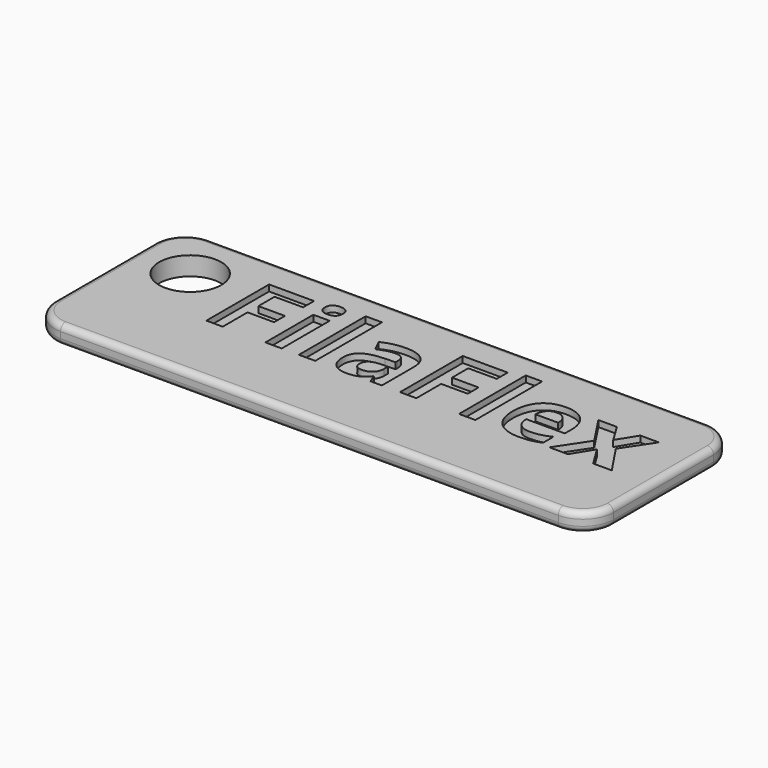
from build123d import *

# Parameters (mm, degrees)
F0_W         = 90
F0_H         = 30
F1_DEPTH     = 3
F2_R         = 1
F3_T1_DEPTH  = 3
F3_T4_ANGLE  = 90
F3_T6_ANGLE  = 90
F3_T8_ANGLE  = 90
F3_T10_ANGLE = 90
F3_T12_ANGLE = 90
F3_T14_ANGLE = 90
F3_T16_ANGLE = 90
F3_T18_ANGLE = 90
F4_R         = 5
F5_DEPTH     = 3
F6_TEXT_SIZE = 17.679558011
F7_DEPTH     = 1


# Not quite as in the source:
# - a fillet or chamfer that OpenCascade refuses, or shapes differently, is made with other operations: its cross-section is extruded or revolved along the edge and cut away or added
# - Text() gives the source's letters only with a copy of the font that has no kerning and outlines rounded to 1/6400 em; it was checked with that copy


with BuildPart() as f1:
    # F0 (on Top) → F1 (new body)
    with BuildSketch(Plane.XY):
        Rectangle(F0_W, F0_H)
    extrude(amount=F1_DEPTH)

    # F2
    f2_edges = [f1.edges().sort_by_distance(p)[0] for p in [
        (0, 15, 3),
        (-45, 0, 3),
        (0, -15, 3),
        (45, 0, 3),
        (0, 15, 0),
        (-45, 0, 0),
        (0, -15, 0),
        (45, 0, 0),
    ]]
    fillet(f2_edges, radius=F2_R)

    # F3: fillet of radius 5 on 4 edges, made by hand

    # F3_s2 → F3_t1 (cut)
    with BuildSketch(Plane.XY):
        with BuildLine():
            ThreePointArc((45.0004, -9.9990343146), (43.5355339059, -13.5355339059), (39.9990343146, -15.0004))
            Line((39.9990343146, -15.0004), (39.9990343146, -15.5005365685))
            ThreePointArc((39.9990343146, -15.5005365685), (42.4995171573, -15.5001365685), (45, -15.5001365685))
            Line((45, -15.5001365685), (45.5001365685, -15))
            ThreePointArc((45.5001365685, -15), (45.5001365685, -12.4995171573), (45.5005365685, -9.9990343146))
            Line((45.5005365685, -9.9990343146), (45.0004, -9.9990343146))
        make_face()
        with BuildLine():
            ThreePointArc((39.9990343146, 15.0004), (43.5355339059, 13.5355339059), (45.0004, 9.9990343146))
            Line((45.0004, 9.9990343146), (45.5005365685, 9.9990343146))
            ThreePointArc((45.5005365685, 9.9990343146), (45.5001365685, 12.4995171573), (45.5001365685, 15))
            Line((45.5001365685, 15), (45, 15.5001365685))
            ThreePointArc((45, 15.5001365685), (42.4995171573, 15.5001365685), (39.9990343146, 15.5005365685))
            Line((39.9990343146, 15.5005365685), (39.9990343146, 15.0004))
        make_face()
        with BuildLine():
            ThreePointArc((-39.9990343146, 15.0004), (-43.5355339059, 13.5355339059), (-45.0004, 9.9990343146))
            Line((-45.0004, 9.9990343146), (-45.5005365685, 9.9990343146))
            ThreePointArc((-45.5005365685, 9.9990343146), (-45.5001365685, 12.4995171573), (-45.5001365685, 15))
            Line((-45.5001365685, 15), (-45, 15.5001365685))
            ThreePointArc((-45, 15.5001365685), (-42.4995171573, 15.5001365685), (-39.9990343146, 15.5005365685))
            Line((-39.9990343146, 15.5005365685), (-39.9990343146, 15.0004))
        make_face()
        with BuildLine():
            ThreePointArc((-45.0004, -9.9990343146), (-43.5355339059, -13.5355339059), (-39.9990343146, -15.0004))
            Line((-39.9990343146, -15.0004), (-39.9990343146, -15.5005365685))
            ThreePointArc((-39.9990343146, -15.5005365685), (-42.4995171573, -15.5001365685), (-45, -15.5001365685))
            Line((-45, -15.5001365685), (-45.5001365685, -15))
            ThreePointArc((-45.5001365685, -15), (-45.5001365685, -12.4995171573), (-45.5005365685, -9.9990343146))
            Line((-45.5005365685, -9.9990343146), (-45.0004, -9.9990343146))
        make_face()
    extrude(amount=F3_T1_DEPTH, mode=Mode.SUBTRACT)

    # F3_s3 → F3_t4 (revolve, cut)
    with BuildSketch(Plane.YZ.offset(-39.9990343146)):
        with BuildLine():
            ThreePointArc((-14.0004, 0), (-14.7075067812, 0.2928932188), (-15.0004, 1))
            Line((-15.0004, 1), (-15.0004, 0))
            Line((-15.0004, 0), (-14.0004, 0))
        make_face()
    revolve(axis=Axis((-39.9990343146, -9.9990343146, 0), (0, 0, -1)), revolution_arc=F3_T4_ANGLE, mode=Mode.SUBTRACT)

    # F3_s5 → F3_t6 (revolve, cut)
    with BuildSketch(Plane.XZ.offset(9.9990343146)):
        with BuildLine():
            ThreePointArc((-44.0004, 3), (-44.7075067812, 2.7071067812), (-45.0004, 2))
            Line((-45.0004, 2), (-45.0004, 3))
            Line((-45.0004, 3), (-44.0004, 3))
        make_face()
    revolve(axis=Axis((-39.9990343146, -9.9990343146, 3), (0, 0, 1)), revolution_arc=F3_T6_ANGLE, mode=Mode.SUBTRACT)

    # F3_s7 → F3_t8 (revolve, cut)
    with BuildSketch(Plane.XZ.offset(-9.9990343146)):
        with BuildLine():
            ThreePointArc((-44.0004, 0), (-44.7075067812, 0.2928932188), (-45.0004, 1))
            Line((-45.0004, 1), (-45.0004, 0))
            Line((-45.0004, 0), (-44.0004, 0))
        make_face()
    revolve(axis=Axis((-39.9990343146, 9.9990343146, 0), (0, 0, -1)), revolution_arc=F3_T8_ANGLE, mode=Mode.SUBTRACT)

    # F3_s9 → F3_t10 (revolve, cut)
    with BuildSketch(Plane.YZ.offset(-39.9990343146)):
        with BuildLine():
            ThreePointArc((14.0004, 3), (14.7075067812, 2.7071067812), (15.0004, 2))
            Line((15.0004, 2), (15.0004, 3))
            Line((15.0004, 3), (14.0004, 3))
        make_face()
    revolve(axis=Axis((-39.9990343146, 9.9990343146, 3), (0, 0, 1)), revolution_arc=F3_T10_ANGLE, mode=Mode.SUBTRACT)

    # F3_s11 → F3_t12 (revolve, cut)
    with BuildSketch(Plane.YZ.offset(39.9990343146)):
        with BuildLine():
            ThreePointArc((14.0004, 0), (14.7075067812, 0.2928932188), (15.0004, 1))
            Line((15.0004, 1), (15.0004, 0))
            Line((15.0004, 0), (14.0004, 0))
        make_face()
    revolve(axis=Axis((39.9990343146, 9.9990343146, 0), (0, 0, -1)), revolution_arc=F3_T12_ANGLE, mode=Mode.SUBTRACT)

    # F3_s13 → F3_t14 (revolve, cut)
    with BuildSketch(Plane.XZ.offset(-9.9990343146)):
        with BuildLine():
            ThreePointArc((44.0004, 3), (44.7075067812, 2.7071067812), (45.0004, 2))
            Line((45.0004, 2), (45.0004, 3))
            Line((45.0004, 3), (44.0004, 3))
        make_face()
    revolve(axis=Axis((39.9990343146, 9.9990343146, 3), (0, 0, 1)), revolution_arc=F3_T14_ANGLE, mode=Mode.SUBTRACT)

    # F3_s15 → F3_t16 (revolve, cut)
    with BuildSketch(Plane.XZ.offset(9.9990343146)):
        with BuildLine():
            ThreePointArc((44.0004, 0), (44.7075067812, 0.2928932188), (45.0004, 1))
            Line((45.0004, 1), (45.0004, 0))
            Line((45.0004, 0), (44.0004, 0))
        make_face()
    revolve(axis=Axis((39.9990343146, -9.9990343146, 0), (0, 0, -1)), revolution_arc=F3_T16_ANGLE, mode=Mode.SUBTRACT)

    # F3_s17 → F3_t18 (revolve, cut)
    with BuildSketch(Plane.YZ.offset(39.9990343146)):
        with BuildLine():
            ThreePointArc((-14.0004, 3), (-14.7075067812, 2.7071067812), (-15.0004, 2))
            Line((-15.0004, 2), (-15.0004, 3))
            Line((-15.0004, 3), (-14.0004, 3))
        make_face()
    revolve(axis=Axis((39.9990343146, -9.9990343146, 3), (0, 0, 1)), revolution_arc=F3_T18_ANGLE, mode=Mode.SUBTRACT)

    # F4 (on face) → F5 (cut)
    with BuildSketch(Plane.XY.offset(3)):
        with Locations((-36, 6)):
            Circle(F4_R)
    extrude(amount=-F5_DEPTH, mode=Mode.SUBTRACT)

    # F6 (on face) → F7 (cut)
    with BuildSketch(Plane.XY.offset(3)):
        with Locations((-28, -2.729281768)):
            Text('FilaFlex', F6_TEXT_SIZE, font='Open Sans', font_style=FontStyle.BOLD, text_align=(TextAlign.LEFT, TextAlign.BOTTOM))
    extrude(amount=-F7_DEPTH, mode=Mode.SUBTRACT)


solid = f1.part
